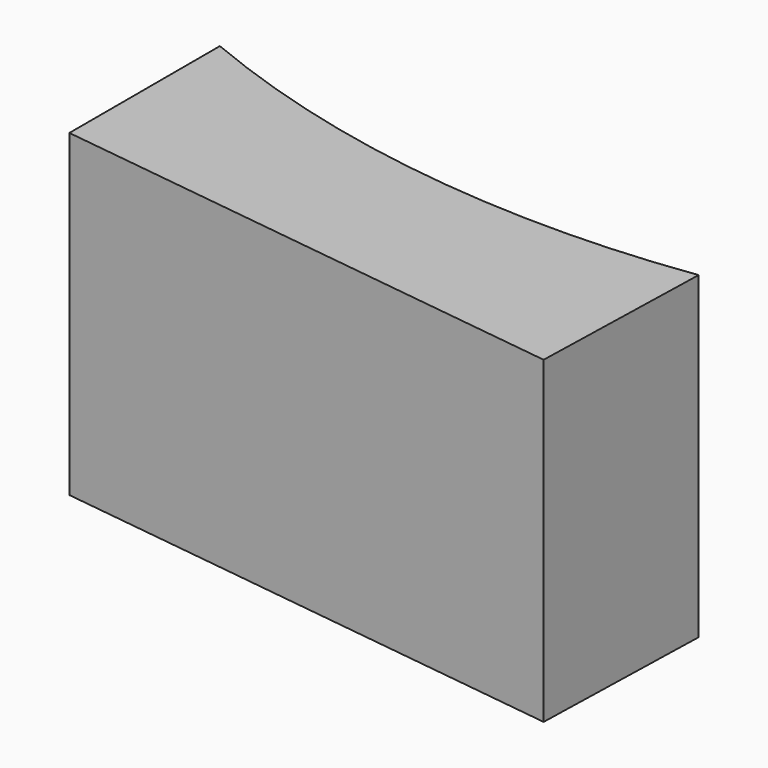
from build123d import *

# Parameters (mm, degrees)
F2_DEPTH = 71.12


# Not quite as in the source:
# - the program builds the solid bodies; features that only make, move or delete a surface that nothing else refers to are left out


with BuildPart() as f2:
    # F0 (on Top) → F2 (new body)
    with BuildSketch(Plane.XY):
        with BuildLine():
            ThreePointArc((31.3367973024, -226.441968581), (-29.2343475788, -226.7229871928), (-87.7529985977, -211.0861701702))
            Line((-87.7529985977, -211.0861701702), (-87.7529985977, -253.0445456505))
            Line((-87.7529985977, -253.0445456505), (30.2124765983, -268.2553707498))
            Line((30.2124765983, -268.2553707498), (31.3367973024, -226.441968581))
        make_face()
    extrude(amount=F2_DEPTH)


solid = f2.part
